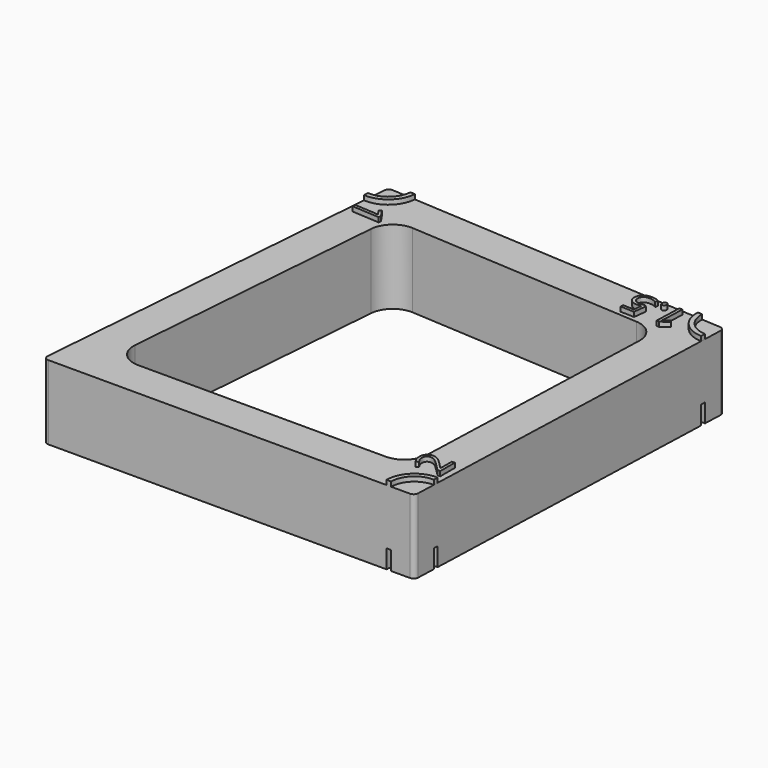
from build123d import *

# Parameters (mm, degrees)
F1_DEPTH     = 20.32
F2_TEXT_SIZE = 10.5833333333
F3_DEPTH     = 1.27
F4_TEXT_SIZE = 10.5833333333
F5_DEPTH     = 5.08
F6_R         = 1.27


# Not quite as in the source:
# - Text() gives the source's letters only with a copy of the font that has no kerning and outlines rounded to 1/6400 em; it was checked with that copy


with BuildPart() as f1:
    # F0 (on Top) → F1 (new body)
    with BuildSketch(Plane.XY):
        Polygon((-101.6, 0), (0, 0), (3.5479501804, 101.6), (-93.1384964557, 107.5135964093), align=None)
        with BuildLine():
            ThreePointArc((-84.2827627479, 90.5421343831), (-82.1183125128, 94.8363249596), (-77.5646794527, 96.3820750952))
            Line((-77.5646794527, 96.3820750952), (-13.1256342678, 92.4408142517))
            ThreePointArc((-13.1256342678, 92.4408142517), (-8.8129073844, 90.3721875089), (-7.1671607423, 85.8810464776))
            Line((-7.1671607423, 85.8810464776), (-9.5973899205, 16.2883881959))
            ThreePointArc((-9.5973899205, 16.2883881959), (-11.5324410197, 11.9421922678), (-15.9435216721, 10.16))
            Line((-15.9435216721, 10.16), (-83.7395826234, 10.16))
            ThreePointArc((-83.7395826234, 10.16), (-88.4025305583, 12.1996152659), (-90.0700076926, 17.0082152579))
            Line((-90.0700076926, 17.0082152579), (-84.2827627479, 90.5421343831))
        make_face(mode=Mode.SUBTRACT)
    extrude(amount=F1_DEPTH)

    # F2 (on face) → F3 (join)
    with BuildSketch(Plane.XY.offset(20.32)):
        with BuildLine():
            Line((-85.5327092918, 107.048406538), (-86.8003404858, 107.1259381833))
            ThreePointArc((-86.8003404858, 107.1259381833), (-88.9725216216, 102.7211905749), (-93.6367117136, 101.1831713401))
            Line((-93.6367117136, 101.1831713401), (-93.7363547652, 99.9170863263))
            ThreePointArc((-93.7363547652, 99.9170863263), (-88.1393266548, 101.762709408), (-85.5327092918, 107.048406538))
        make_face()
        with BuildLine():
            Line((-2.7902057896, 101.987658226), (-4.0578369836, 102.0651898713))
            ThreePointArc((-4.0578369836, 102.0651898713), (-2.0925119511, 96.4765649273), (3.2820160155, 93.9846418981))
            Line((3.2820160155, 93.9846418981), (3.3263383763, 95.2538682484))
            ThreePointArc((3.3263383763, 95.2538682484), (-1.1524349292, 97.3304707728), (-2.7902057896, 101.987658226))
        make_face()
        with BuildLine():
            Line((0.2216118041, 6.3461317516), (0.2659341649, 7.6153581019))
            ThreePointArc((0.2659341649, 7.6153581019), (-5.2932967829, 5.4813692786), (-7.62, 0))
            Line((-7.62, 0), (-6.35, 0))
            ThreePointArc((-6.35, 0), (-4.4110806524, 4.5678077322), (0.2216118041, 6.3461317516))
        make_face()
        with Locations(Location((-92.2019572971, 98.0334979576), (0, 0, -93.5))):
            Text('1', F2_TEXT_SIZE, font='Open Sans', text_align=(TextAlign.LEFT, TextAlign.BOTTOM))
        with Locations(Location((-4.6325196969, 100.9892123891), (0, 0, 178))):
            Text('1.5', F2_TEXT_SIZE, font='Open Sans', text_align=(TextAlign.LEFT, TextAlign.BOTTOM))
        with Locations(Location((-1.1785078296, 9.7975186866), (0, 0, 90))):
            Text('2', F2_TEXT_SIZE, font='Open Sans', text_align=(TextAlign.LEFT, TextAlign.BOTTOM))
    extrude(amount=F3_DEPTH)

    # F4 (on face) → F5 (cut)
    with BuildSketch(Plane(origin=(0, 0, 0), x_dir=(1, 0, 0), z_dir=(0, 0, -1))):
        with BuildLine():
            Line((0.2659341649, -7.6153581019), (0.2216118041, -6.3461317516))
            ThreePointArc((0.2216118041, -6.3461317516), (-4.4110806524, -4.5678077322), (-6.35, 0))
            Line((-6.35, 0), (-7.62, 0))
            ThreePointArc((-7.62, 0), (-5.2932967829, -5.4813692786), (0.2659341649, -7.6153581019))
        make_face()
        with BuildLine():
            ThreePointArc((-93.6367117136, -101.1831713401), (-88.9725216216, -102.7211905749), (-86.8003404858, -107.1259381833))
            Line((-86.8003404858, -107.1259381833), (-85.5327092918, -107.048406538))
            ThreePointArc((-85.5327092918, -107.048406538), (-88.1393266548, -101.762709408), (-93.7363547652, -99.9170863263))
            Line((-93.7363547652, -99.9170863263), (-93.6367117136, -101.1831713401))
        make_face()
        with BuildLine():
            ThreePointArc((-2.7902057896, -101.987658226), (-1.1524349292, -97.3304707728), (3.3263383763, -95.2538682484))
            Line((3.3263383763, -95.2538682484), (3.2820160155, -93.9846418981))
            ThreePointArc((3.2820160155, -93.9846418981), (-2.0925119511, -96.4765649273), (-4.0578369836, -102.0651898713))
            Line((-4.0578369836, -102.0651898713), (-2.7902057896, -101.987658226))
        make_face()
        with Locations(Location((-92.5652930444, -94.6246250269), (0, 0, -85.5))):
            Text('1', F4_TEXT_SIZE, font='Open Sans', text_align=(TextAlign.LEFT, TextAlign.BOTTOM))
        with Locations(Location((-19.3834110437, -101.9785894583), (0, 0, 3.5))):
            Text('1.5', F4_TEXT_SIZE, font='Open Sans', text_align=(TextAlign.LEFT, TextAlign.BOTTOM))
        with Locations(Location((-0.8413404204, -14.3434358912), (0, 0, 92))):
            Text('2', F4_TEXT_SIZE, font='Open Sans', text_align=(TextAlign.LEFT, TextAlign.BOTTOM))
    extrude(amount=-F5_DEPTH, mode=Mode.SUBTRACT)

    # F6
    f6_edges = [f1.edges().sort_by_distance(p)[0] for p in [
        (-101.6, 0, 10.16),
        (-93.138496, 107.513596, 10.16),
        (3.54795, 101.6, 10.16),
        (0, 0, 10.16),
    ]]
    fillet(f6_edges, radius=F6_R)


solid = f1.part
